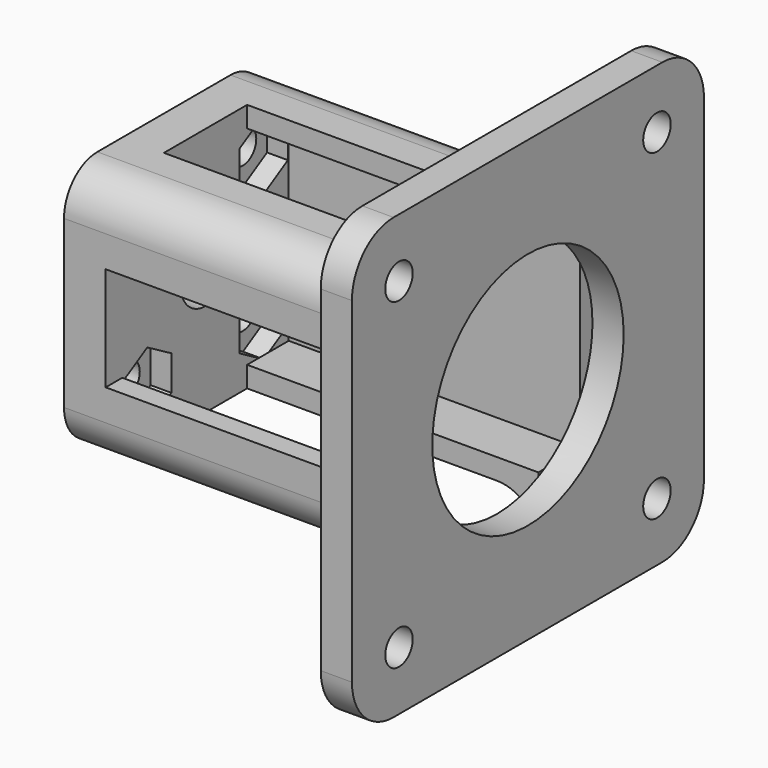
from build123d import *

# Parameters (mm, degrees)
F0_W     = 24
F0_H     = 24
F0_R     = 1.6
F0_R_2   = 3
F1_DEPTH = 4
F4_DEPTH = 2
F5_DEPTH = 28
F6_W     = 42.3
F6_H     = 42.3
F6_R     = 1.65
F6_R_2   = 11.5
F7_DEPTH = 3
F8_R     = 5
F9_F1_R  = 4
F9_F2_R  = 4


with BuildPart() as f1:
    # F0 (on Right) → F1 (new body)
    with BuildSketch(Plane.YZ):
        Rectangle(F0_W, F0_H)
        with Locations((-7, -7)):
            Circle(F0_R, mode=Mode.SUBTRACT)
        with Locations((7, -7)):
            Circle(F0_R, mode=Mode.SUBTRACT)
        with Locations((-7, 7)):
            Circle(F0_R, mode=Mode.SUBTRACT)
        Circle(F0_R_2, mode=Mode.SUBTRACT)
        with Locations((7, 7)):
            Circle(F0_R, mode=Mode.SUBTRACT)
    extrude(amount=F1_DEPTH)

    # F2 (on face) → F4 (cut)
    with BuildSketch(Plane.YZ.offset(4)):
        Polygon((7, -3.6513684387), (4.1, -5.3256842194), (4.1, -8.6743157806), (7, -10.3486315613), (9.9, -8.6743157806), (9.9, -5.3256842194), align=None)
        Polygon((4.1, 5.3256842194), (7, 3.6513684387), (9.9, 5.3256842194), (9.9, 8.6743157806), (7, 10.3486315613), (4.1, 8.6743157806), align=None)
        Polygon((-9.9, 5.3256842194), (-7, 3.6513684387), (-4.1, 5.3256842194), (-4.1, 8.6743157806), (-7, 10.3486315613), (-9.9, 8.6743157806), align=None)
        Polygon((-4.1, -5.3256842194), (-7, -3.6513684387), (-9.9, -5.3256842194), (-9.9, -8.6743157806), (-7, -10.3486315613), (-4.1, -8.6743157806), align=None)
    extrude(amount=-F4_DEPTH, mode=Mode.SUBTRACT)

    # F3 (on face) → F5 (join)
    with BuildSketch(Plane.YZ.offset(4)):
        Polygon((-5, 12), (-12, 12), (-12, 5), (-10, 5), (-10, 10), (-5, 10), align=None)
        Polygon((12, 12), (5, 12), (5, 10), (10, 10), (10, -10), (5, -10), (5, -12), (12, -12), align=None)
        Polygon((-10, -5), (-12, -5), (-12, -12), (-5, -12), (-5, -10), (-10, -10), align=None)
    extrude(amount=F5_DEPTH)

    # F6 (on face) → F7 (join)
    with BuildSketch(Plane.YZ.offset(32)):
        Rectangle(F6_W, F6_H)
        with Locations((-15.5, -15.5)):
            Circle(F6_R, mode=Mode.SUBTRACT)
        with Locations((15.5, -15.5)):
            Circle(F6_R, mode=Mode.SUBTRACT)
        with Locations((-15.5, 15.5)):
            Circle(F6_R, mode=Mode.SUBTRACT)
        Circle(F6_R_2, mode=Mode.SUBTRACT)
        with Locations((15.5, 15.5)):
            Circle(F6_R, mode=Mode.SUBTRACT)
    extrude(amount=F7_DEPTH)

    # F8
    f8_edges = [f1.edges().sort_by_distance(p)[0] for p in [
        (33.5, 21.15, 21.15),
        (33.5, 21.15, -21.15),
        (33.5, -21.15, -21.15),
        (33.5, -21.15, 21.15),
    ]]
    fillet(f8_edges, radius=F8_R)

    # F9: fillet of radius 4 on 7 edges, made by hand

    # F9_f1
    f9_f1_edges = [f1.edges().sort_by_distance(p)[0] for p in [
        (16, 12, 12),
        (16, 12, -12),
        (16, -12, -12),
        (16, -12, 12),
    ]]
    fillet(f9_f1_edges, radius=F9_F1_R)

    # F9_f2
    f9_f2_edges = [f1.edges().sort_by_distance(p)[0] for p in [
        (32, 12, 0),
        (32, -6.5, -12),
        (32, -12, 6.5),
        (32, -10.8284271247, 10.8284271247),
        (32, -10.8284271247, -10.8284271247),
        (32, 10.8284271247, -10.8284271247),
        (32, 10.8284271247, 10.8284271247),
    ]]
    fillet(f9_f2_edges, radius=F9_F2_R)


solid = f1.part
